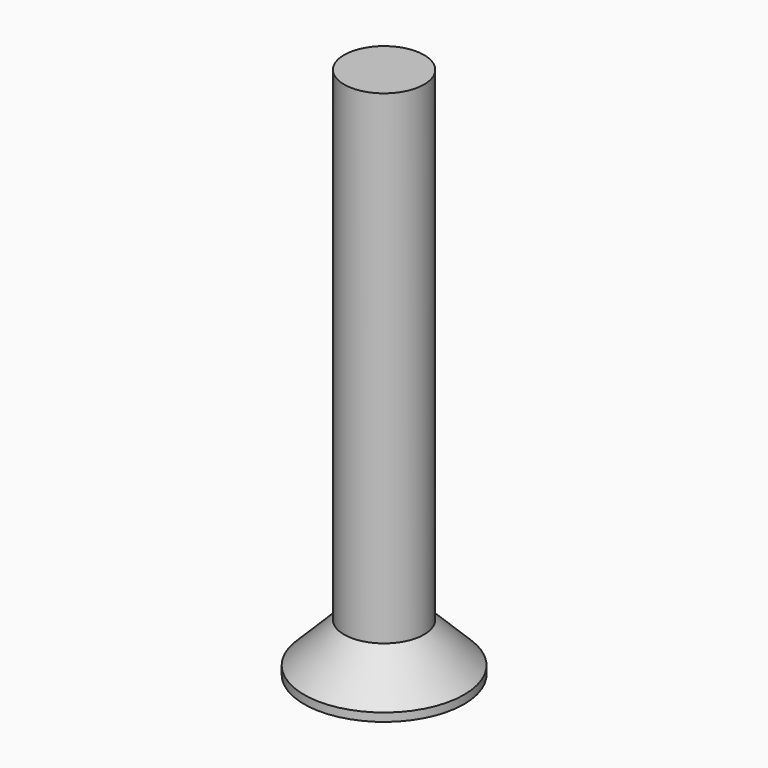
from build123d import *

# Parameters (mm, degrees)
F0_R        = 1.45
F1_DEPTH    = 17.5
F2_R        = 2.9
F3_DEPTH    = 1.8
F4_W        = 1
F4_H        = 1
F5_DEPTH    = 1.5
F6_S5_R     = 1.45
F6_T6_DEPTH = 6


# Not quite as in the source:
# - a fillet or chamfer that OpenCascade refuses, or shapes differently, is made with other operations: its cross-section is extruded or revolved along the edge and cut away or added


with BuildPart() as f1:
    # F0 (on Top) → F1 (new body)
    with BuildSketch(Plane.XY):
        Circle(F0_R)
    extrude(amount=F1_DEPTH)

    # F2 (on Top) → F3 (join)
    with BuildSketch(Plane.XY):
        Circle(F2_R)
    extrude(amount=-F3_DEPTH)

    # F4 (on face) → F5 (cut)
    with BuildSketch(Plane(origin=(0, 0, -1.8), x_dir=(1, 0, 0), z_dir=(0, 0, -1))):
        with Locations((1, 0)):
            Rectangle(F4_W, F4_H)
        Rectangle(F4_W, F4_H)
        with Locations((0, 1)):
            Rectangle(F4_W, F4_H)
        with Locations((-1, 0)):
            Rectangle(F4_W, F4_H)
        with Locations((0, -1)):
            Rectangle(F4_W, F4_H)
    extrude(amount=-F5_DEPTH, mode=Mode.SUBTRACT)

    # F6: chamfer of 1.5 on 1 edges, made by hand


with BuildPart() as f6_tool2:
    # F6_s3 → F6_t4 (revolve)
    with BuildSketch(Plane.XZ):
        Polygon((2.9, -1.5), (1.4, 0), (2.9, 0), align=None)
    revolve(axis=Axis((0, 0, 0), (0, 0, 1)))

    # F6_s5 → F6_t6 (cut, symmetric)
    with BuildSketch(Plane.XY.offset(-0.7)):
        Circle(F6_S5_R)
    extrude(amount=F6_T6_DEPTH, both=True, mode=Mode.SUBTRACT)


with BuildPart() as f1_1:
    add(f1.part)

    # F6_t1: cut F6_tool2
    add(f6_tool2.part, mode=Mode.SUBTRACT)


solid = f1_1.part
